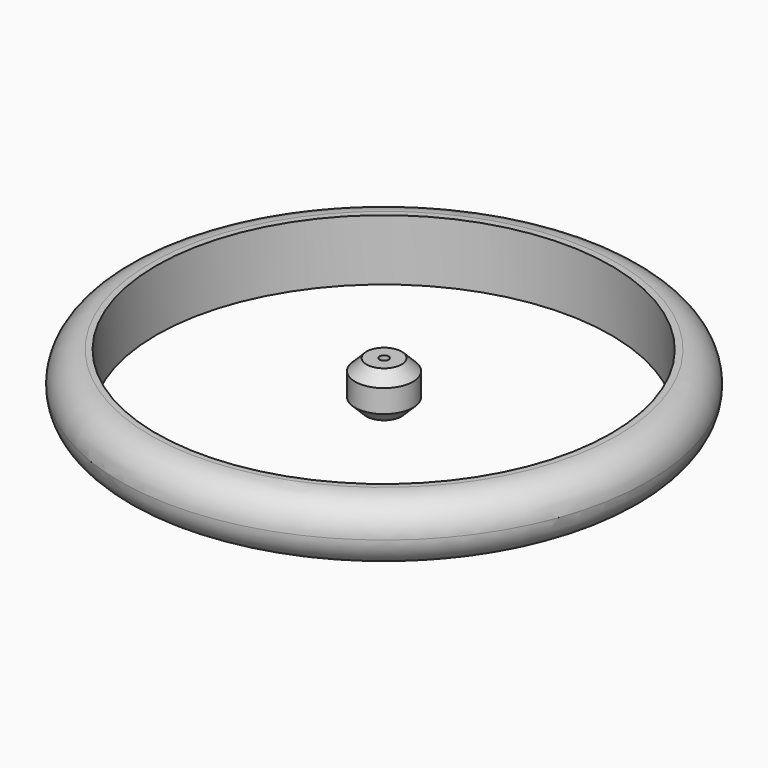
from build123d import *

# Parameters (mm, degrees)
F0_R     = 346
F0_R_2   = 298
F1_DEPTH = 80
F2_R     = 39.99999
F0_R_3   = 38
F0_R_4   = 6
F3_DEPTH = 70
F4_DEPTH = 10
F5_SIZE  = 15


# Not quite as in the source:
# - a fillet or chamfer is up to 0.001 mm smaller than in the source, because OpenCascade refuses the exact size


with BuildPart() as f1:
    # F0 (on Top) → F1 (new body)
    with BuildSketch(Plane.XY):
        Circle(F0_R)
        with Locations((0, -0.6947662914)):
            Circle(F0_R_2, mode=Mode.SUBTRACT)
    extrude(amount=-F1_DEPTH)

    # F2 (radius 40 in the source; OpenCascade refuses exactly that, so slightly less here)
    f2_edges = [f1.edges().sort_by_distance(p)[0] for p in [
        (-346, 0, 0),
        (-346, 0, -80),
    ]]
    fillet(f2_edges, radius=F2_R)


with BuildPart() as f3:
    # F0 (on Top) → F3 (new body)
    with BuildSketch(Plane.XY):
        Circle(F0_R_3)
        Circle(F0_R_4, mode=Mode.SUBTRACT)
    extrude(amount=-F3_DEPTH)

    # F4 (cut): a face of the model
    f4_faces = [f3.faces().sort_by_distance(p)[0] for p in [
        (-36.9251976926, 0, 0),
    ]]
    extrude(f4_faces, amount=-F4_DEPTH, mode=Mode.SUBTRACT)

    # F5
    f5_edges = [f3.edges().sort_by_distance(p)[0] for p in [
        (-38, 0, -10),
        (-38, 0, -70),
    ]]
    chamfer(f5_edges, length=F5_SIZE)


solid = Compound([f1.part, f3.part])
